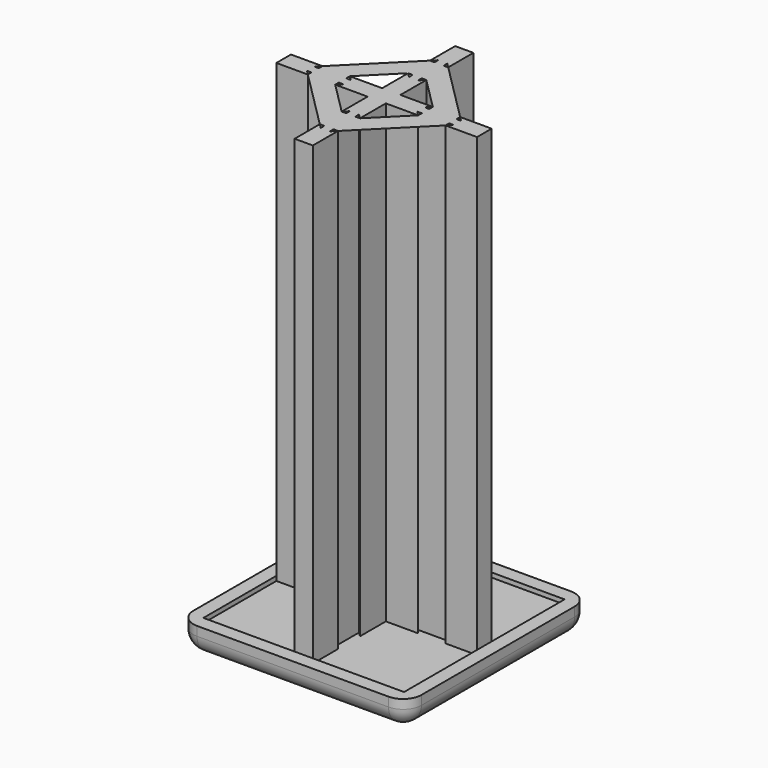
from build123d import *

# Parameters (mm, degrees)
F0_W     = 5.08
F0_H     = 5.08
F1_DEPTH = 127
F2_W     = 55.88
F2_H     = 55.88
F3_DEPTH = 2.54
F4_W     = 63.5
F4_H     = 63.5
F4_W_2   = 55.88
F4_H_2   = 55.88
F5_DEPTH = 3.81
F6_DEPTH = 3.81
F7_R     = 5.08


with BuildPart() as f1:
    # F0 (on Top) → F1 (new body)
    with BuildSketch(Plane.XY):
        Polygon((2.54, -2.54), (-2.54, -2.54), (-2.54, -11.557), (-1.27, -10.287), (-1.27, -15.367), (-1.27, -20.447), (-2.54, -19.177), (-2.54, -27.94), (2.54, -27.94), (2.54, -19.177), (1.27, -20.447), (1.27, -15.367), (1.27, -10.287), (2.54, -11.557), align=None)
        Rectangle(F0_W, F0_H)
        Polygon((-2.54, -2.54), (-2.54, 2.54), (-11.557, 2.54), (-10.287, 1.27), (-15.367, 1.27), (-20.447, 1.27), (-19.177, 2.54), (-27.94, 2.54), (-27.94, -2.54), (-19.177, -2.54), (-20.447, -1.27), (-15.367, -1.27), (-10.287, -1.27), (-11.557, -2.54), align=None)
        Polygon((2.54, 27.94), (-2.54, 27.94), (-2.54, 19.177), (-1.27, 20.447), (-1.27, 15.367), (-1.27, 10.287), (-2.54, 11.557), (-2.54, 2.54), (2.54, 2.54), (2.54, 11.557), (1.27, 10.287), (1.27, 15.367), (1.27, 20.447), (2.54, 19.177), align=None)
        Polygon((11.557, 2.54), (2.54, 2.54), (2.54, -2.54), (11.557, -2.54), (10.287, -1.27), (15.367, -1.27), (20.447, -1.27), (19.177, -2.54), (27.94, -2.54), (27.94, 2.54), (19.177, 2.54), (20.447, 1.27), (15.367, 1.27), (10.287, 1.27), align=None)
    extrude(amount=F1_DEPTH)

    # F2 (on face) → F3 (join)
    with BuildSketch(Plane(origin=(0, 0, 0), x_dir=(1, 0, 0), z_dir=(0, 0, -1))):
        Rectangle(F2_W, F2_H)
    extrude(amount=F3_DEPTH)


with BuildPart() as f5:
    # F4 (on face) → F5 (new body)
    with BuildSketch(Plane(origin=(0, 0, -2.54), x_dir=(1, 0, 0), z_dir=(0, 0, -1))):
        Rectangle(F4_W, F4_H)
        Rectangle(F4_W_2, F4_H_2, mode=Mode.SUBTRACT)
        Rectangle(F4_W_2, F4_H_2)
    extrude(amount=F5_DEPTH)

    # F4 (on face) → F6 (join)
    with BuildSketch(Plane(origin=(0, 0, -2.54), x_dir=(1, 0, 0), z_dir=(0, 0, -1))):
        Rectangle(F4_W, F4_H)
        Rectangle(F4_W_2, F4_H_2, mode=Mode.SUBTRACT)
    extrude(amount=-F6_DEPTH)

    # F7
    f7_edges = [f5.edges().sort_by_distance(p)[0] for p in [
        (-31.75, -31.75, -2.54),
        (31.75, -31.75, -2.54),
        (31.75, 31.75, -2.54),
        (31.75, 0, -6.35),
        (0, -31.75, -6.35),
        (-31.75, 31.75, -2.54),
        (0, 31.75, -6.35),
        (-31.75, 0, -6.35),
    ]]
    fillet(f7_edges, radius=F7_R)


solid = Compound([f1.part, f5.part])
